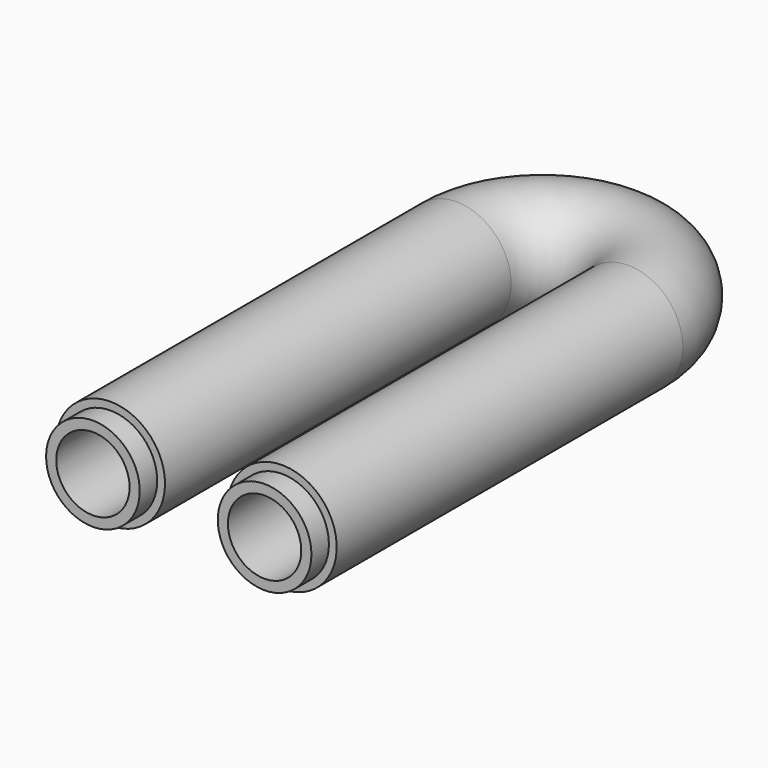
from build123d import *

# Parameters (mm, degrees)
F1_R     = 8.89
F1_R_2   = 5.969
F3_DEPTH = 3.556
F5_R     = 8.89
F5_R_2   = 7.62
F7_DEPTH = 3.556


# Not quite as in the source:
# - a feature of the source that left no trace in its solid (it failed there, or was rolled back) is left out
# - a pattern or mirror of a feature is missing from the dataset's text; its kind, count and spacing are read off the source's solid


with BuildPart() as f2:
    # F2: sweep along a path in F0
    with BuildLine(Plane.XY) as f2_path:
        Line((0, 0), (0, 70.4088))
        ThreePointArc((0, 70.4088), (13.97, 84.3788), (27.94, 70.4088))
        Line((27.94, 70.4088), (27.94, 0))
        Line((27.94, 0), (27.94, -3.556))
    # F1 (on Front) → F2 (sweep)
    with BuildSketch(Plane.XZ):
        Circle(F1_R)
        Circle(F1_R_2, mode=Mode.SUBTRACT)
    sweep(path=f2_path.line)

    # F3 (add): a face of the model
    f3_faces = [f2.faces().sort_by_distance(p)[0] for p in [
        (-8.6385528286, 0, 0),
    ]]
    extrude(f3_faces, amount=F3_DEPTH)

    # F5 (on face) → F7 (cut)
    with BuildSketch(Plane.XZ.offset(3.556)):
        with Locations((27.94, 0)):
            Circle(F5_R)
        with Locations((27.94, 0)):
            Circle(F5_R_2, mode=Mode.SUBTRACT)
    f7 = extrude(amount=-F7_DEPTH, mode=Mode.SUBTRACT)

    # F7_copies: F7 across plane
    add(f7.mirror(Plane(origin=(13.97, 0, 0), x_dir=(0, 0, -1), z_dir=(-1, 0, 0))), mode=Mode.SUBTRACT)


solid = f2.part
